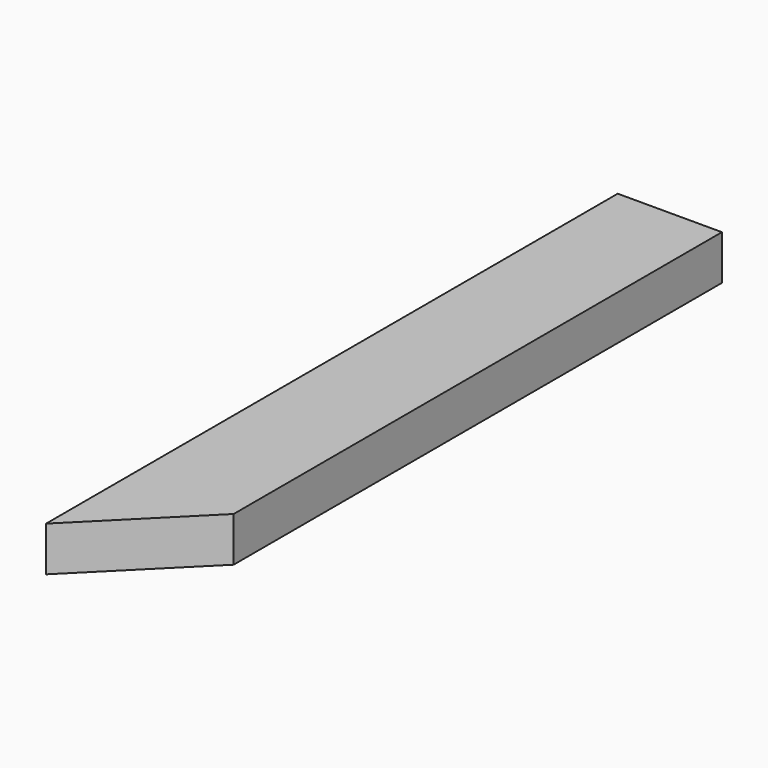
from build123d import *

# Parameters (mm, degrees)
F0_W     = 88.9
F0_H     = 38.1
F1_DEPTH = 304.8
F2_SIZE2 = 88.89999
F2_SIZE  = 88.89999


# Not quite as in the source:
# - a fillet or chamfer is up to 0.001 mm smaller than in the source, because OpenCascade refuses the exact size


with BuildPart() as f1:
    # F0 (on Front) → F1 (new body, symmetric)
    with BuildSketch(Plane.XZ):
        Rectangle(F0_W, F0_H)
    extrude(amount=F1_DEPTH, both=True)

    # F2 (size 88.9 and 88.9 in the source; OpenCascade refuses exactly that, so slightly less here)
    f2_edges = [f1.edges().sort_by_distance(p)[0] for p in [
        (44.45, -304.8, 0),
    ]]
    chamfer(f2_edges, length=F2_SIZE, length2=F2_SIZE2)


solid = f1.part
